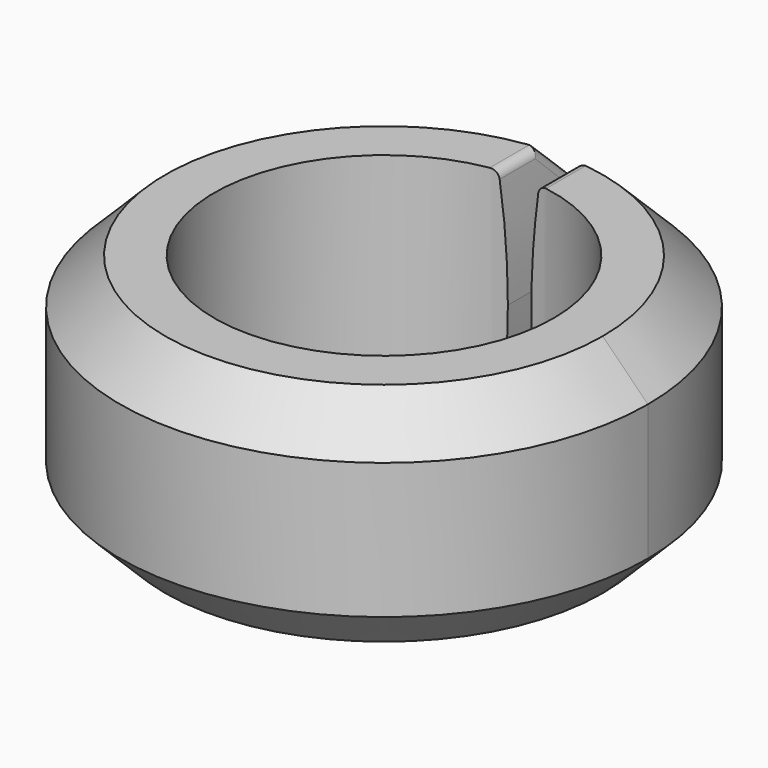
from build123d import *

# Parameters (mm, degrees)
F1_DEPTH = 19.05
F2_SIZE  = 3.81
F4_DEPTH = 25.4
F5_R     = 0.762


with BuildPart() as f1:
    # F0 (on Top) → F1 (new body)
    with BuildSketch(Plane.XY):
        with BuildLine():
            ThreePointArc((0.8676202269, 14.2685876747), (10.4102819289, 9.7964988261), (14.2949417309, 0))
            ThreePointArc((14.2949417309, 0), (-9.7964988261, -10.4102819289), (-0.8676202269, 14.2685876747))
            Line((-0.8676202269, 14.2685876747), (-0.8676202269, 22.2080584505))
            ThreePointArc((-0.8676202269, 22.2080584505), (-15.4056445087, -16.019261602), (22.225, 0))
            ThreePointArc((22.225, 0), (16.019261602, 15.4056445087), (0.8676202269, 22.2080584505))
            Line((0.8676202269, 22.2080584505), (0.8676202269, 14.2685876747))
        make_face()
    extrude(amount=F1_DEPTH)

    # F2
    f2_edges = [f1.edges().sort_by_distance(p)[0] for p in [
        (-15.405645, -16.019262, 19.05),
        (-15.405645, -16.019262, 0),
    ]]
    chamfer(f2_edges, length=F2_SIZE)

    # F3 (on Front) → F4 (cut)
    with BuildSketch(Plane.XZ):
        with BuildLine():
            ThreePointArc((2.6717553826, -5.5055550528), (0.9808079105, 9.7828422745), (2.9202771279, 25.0417038096))
            Line((2.9202771279, 25.0417038096), (-2.9202771279, 25.0417038096))
            ThreePointArc((-2.9202771279, 25.0417038096), (-1.465879157, 17.2066583018), (-0.9786513266, 9.2526768707))
            ThreePointArc((-0.9786513266, 9.2526768707), (-1.4033109655, 1.8251602795), (-2.6717553826, -5.5055550528))
            Line((-2.6717553826, -5.5055550528), (2.6717553826, -5.5055550528))
        make_face()
    extrude(amount=-F4_DEPTH, mode=Mode.SUBTRACT)

    # F5
    f5_edges = [f1.edges().sort_by_distance(p)[0] for p in [
        (-1.45887, 20.2631, 17.149451),
        (1.45887, 20.2631, 17.149451),
        (-0.979225, 22.203417, 9.526057),
        (0.979225, 22.203417, 9.526057),
        (1.719324, 16.262865, 19.05),
        (-1.719324, 16.262865, 19.05),
        (-1.394665, 20.267988, 1.900916),
        (-1.638853, 16.271309, 0),
        (1.394665, 20.267988, 1.900916),
        (1.638853, 16.271309, 0),
    ]]
    fillet(f5_edges, radius=F5_R)


solid = f1.part
